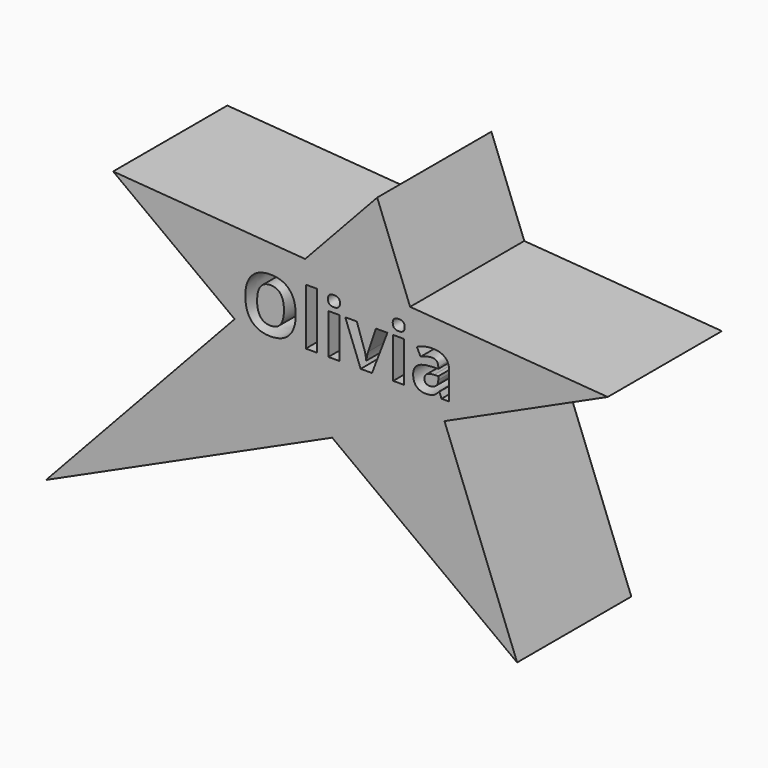
from build123d import *

# Parameters (mm, degrees)
F1_DEPTH     = 9.525
F2_TEXT_SIZE = 4.9465542866
F3_DEPTH     = 6.35


# Not quite as in the source:
# - Text() gives the source's letters only with a copy of the font that has no kerning and outlines rounded to 1/6400 em; it was checked with that copy


with BuildPart() as f1:
    # F0 (on Front) → F1 (new body)
    with BuildSketch(Plane.XZ):
        Polygon((-39.0288941294, 44.035166035), (-51.6148433089, 30.4933227599), (-32.5192062817, 39.1861131853), (-20.1751549052, 29.9910551573), (-25.0240188114, 42.5981016823), (-14.127640985, 47.5583933294), (-27.3187858301, 48.5644961055), (-29.5141786337, 54.2725175619), (-34.3227869468, 49.0986987884), (-47.1387580037, 50.076186657), align=None)
    extrude(amount=F1_DEPTH)

    # F2 (on face) → F3 (cut)
    with BuildSketch(Plane.XZ.offset(9.525)):
        with Locations((-38.6035181582, 43.8474677503)):
            Text('Olivia', F2_TEXT_SIZE, font='Open Sans', font_style=FontStyle.BOLD, text_align=(TextAlign.LEFT, TextAlign.BOTTOM))
    extrude(amount=-F3_DEPTH, mode=Mode.SUBTRACT)


solid = f1.part
